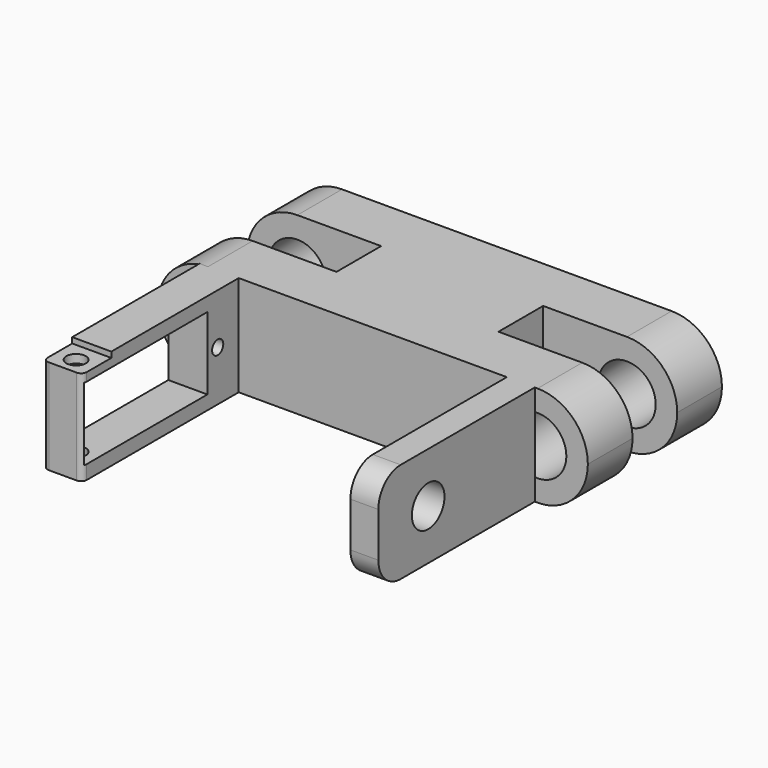
from build123d import *

# Parameters (mm, degrees)
F0_R         = 5.15
F1_DEPTH     = 30
F2_W         = 26.2453191746
F2_H         = 10
F2_W_2       = 30.2312795687
F3_DEPTH     = 25
F4_W         = 5
F4_H         = 18
F4_W_2       = 7
F5_DEPTH     = 35
F6_W         = 27.5
F6_H         = 13
F6_R         = 1.25
F7_DEPTH     = 25
F8_R         = 3.65
F9_DEPTH     = 25
F10_R        = 5
F11_R        = 1.75
F12_DEPTH    = 25
F13_W        = 7
F13_H        = 6.5
F14_DEPTH    = 1
F15_T1_DEPTH = 22


# Not quite as in the source:
# - a fillet or chamfer that OpenCascade refuses, or shapes differently, is made with other operations: its cross-section is extruded or revolved along the edge and cut away or added


with BuildPart() as f1:
    # F0 (on Front) → F1 (new body)
    with BuildSketch(Plane.XZ):
        with BuildLine():
            ThreePointArc((-59, -9), (-52.6360389693, -6.3639610307), (-50, 0))
            ThreePointArc((-50, 0), (-52.6360389693, 6.3639610307), (-59, 9))
            ThreePointArc((-59, 9), (-68, 0), (-59, -9))
        make_face()
        with Locations((-59, 0)):
            Circle(F0_R, mode=Mode.SUBTRACT)
        with BuildLine():
            ThreePointArc((-59, 9), (-52.6360389693, 6.3639610307), (-50, 0))
            ThreePointArc((-50, 0), (-52.6360389693, -6.3639610307), (-59, -9))
            Line((-59, -9), (0, -9))
            ThreePointArc((0, -9), (-9, 0), (0, 9))
            Line((0, 9), (-59, 9))
        make_face()
        with BuildLine():
            ThreePointArc((9, 0), (6.3639610307, 6.3639610307), (0, 9))
            ThreePointArc((0, 9), (-9, 0), (0, -9))
            ThreePointArc((0, -9), (6.3639610307, -6.3639610307), (9, 0))
        make_face()
        Circle(F0_R, mode=Mode.SUBTRACT)
    extrude(amount=F1_DEPTH)

    # F2 (on face) → F3 (cut)
    with BuildSketch(Plane.XY.offset(9)):
        with Locations((-1.8773404127, -15)):
            Rectangle(F2_W, F2_H)
        with Locations((-59.1156397844, -15)):
            Rectangle(F2_W_2, F2_H)
    extrude(amount=-F3_DEPTH, mode=Mode.SUBTRACT)

    # F4 (on face) → F5 (join)
    with BuildSketch(Plane.XZ.offset(30)):
        with Locations((-3, 0)):
            Rectangle(F4_W, F4_H)
        with Locations((-57, 0)):
            Rectangle(F4_W_2, F4_H)
    extrude(amount=F5_DEPTH)

    # F6 (on face) → F7 (cut)
    with BuildSketch(Plane(origin=(-60.5, 0, 0), x_dir=(0, -1, 0), z_dir=(-1, 0, 0))):
        with Locations((50.75, 0)):
            Rectangle(F6_W, F6_H)
        with Locations((34.7, 0)):
            Circle(F6_R)
    extrude(amount=-F7_DEPTH, mode=Mode.SUBTRACT)

    # F8 (on face) → F9 (cut)
    with BuildSketch(Plane(origin=(-5.5, 0, 0), x_dir=(0, -1, 0), z_dir=(-1, 0, 0))):
        with Locations((53.85, 0)):
            Circle(F8_R)
    extrude(amount=-F9_DEPTH, mode=Mode.SUBTRACT)

    # F10
    f10_edges = [f1.edges().sort_by_distance(p)[0] for p in [
        (-3, -65, 9),
        (-3, -65, -9),
    ]]
    fillet(f10_edges, radius=F10_R)

    # F11 (on face) → F12 (cut)
    with BuildSketch(Plane.XY.offset(9)):
        with Locations((-57, -62)):
            Circle(F11_R)
    extrude(amount=-F12_DEPTH, mode=Mode.SUBTRACT)

    # F13 (on face) → F14 (cut)
    with BuildSketch(Plane.XY.offset(9)):
        with Locations((-57, -61.75)):
            Rectangle(F13_W, F13_H)
    extrude(amount=-F14_DEPTH, mode=Mode.SUBTRACT)

    # F15: fillet of radius 1 on 2 edges, made by hand

    # F15_s2 → F15_t1 (cut)
    with BuildSketch(Plane.XY.offset(-11.5)):
        with BuildLine():
            ThreePointArc((-59.5, -65), (-60.2071067812, -64.7071067812), (-60.5, -64))
            Line((-60.5, -64), (-60.5, -65))
            Line((-60.5, -65), (-59.5, -65))
        make_face()
        with BuildLine():
            ThreePointArc((-53.5, -64), (-53.7928932188, -64.7071067812), (-54.5, -65))
            Line((-54.5, -65), (-53.5, -65))
            Line((-53.5, -65), (-53.5, -64))
        make_face()
    extrude(amount=F15_T1_DEPTH, mode=Mode.SUBTRACT)


solid = f1.part
